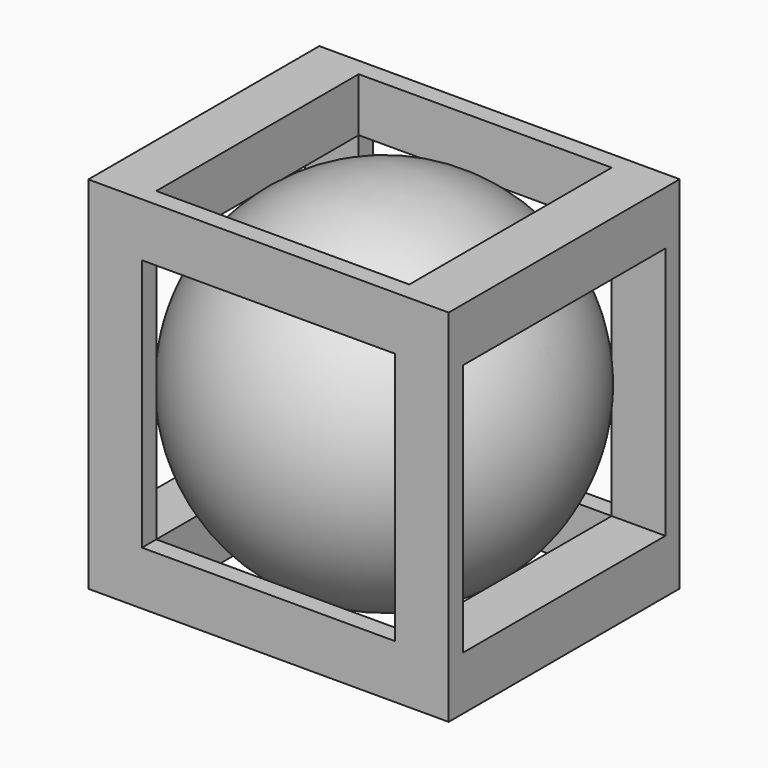
from build123d import *

# Parameters (mm, degrees)
F4_W          = 100.7106781187
F4_H          = 100.7106781187
F5_DEPTH      = 40.3553390593
F5_DEPTH_BACK = 40.3553390593
F6_W          = 70.7106781187
F6_H          = 70.7106781187
F7_DEPTH      = 100.7116781187
F8_W          = 70.7106781187
F8_H          = 70.7106781187
F9_DEPTH      = 80.7106781187
F10_W         = 70.7106781187
F10_H         = 70.7106781187
F11_DEPTH     = 100.7106781187


with BuildPart() as f3:
    # F2 (on Front) → F3 (revolve)
    with BuildSketch(Plane.XZ):
        with BuildLine():
            Line((-50, 0), (50, 0))
            ThreePointArc((50, 0), (0, 50), (-50, 0))
        make_face()
    revolve(axis=Axis((33.0418199301, 0, 0), (1, 0, 0)))


with BuildPart() as f5:
    # F4 (on Front) → F5 (new body, two sides)
    with BuildSketch(Plane.XZ) as f5_sk:
        Rectangle(F4_W, F4_H)
    extrude(amount=F5_DEPTH)
    extrude(f5_sk.sketch, amount=-F5_DEPTH_BACK)

    # F6 (on face) → F7 (cut, through all)
    with BuildSketch(Plane(origin=(-50.3553390593, 0, 0), x_dir=(0, -1, 0), z_dir=(-1, 0, 0))):
        Rectangle(F6_W, F6_H)
    extrude(amount=-F7_DEPTH, mode=Mode.SUBTRACT)

    # F8 (on face) → F9 (cut, through all)
    with BuildSketch(Plane(origin=(0, 40.3553390593, 0), x_dir=(-1, 0, 0), z_dir=(0, 1, 0))):
        Rectangle(F8_W, F8_H)
    extrude(amount=-F9_DEPTH, mode=Mode.SUBTRACT)

    # F10 (on face) → F11 (cut, through all)
    with BuildSketch(Plane(origin=(0, 0, -50.3553390593), x_dir=(1, 0, 0), z_dir=(0, 0, -1))):
        Rectangle(F10_W, F10_H)
    extrude(amount=-F11_DEPTH, mode=Mode.SUBTRACT)


solid = Compound([f3.part, f5.part])
